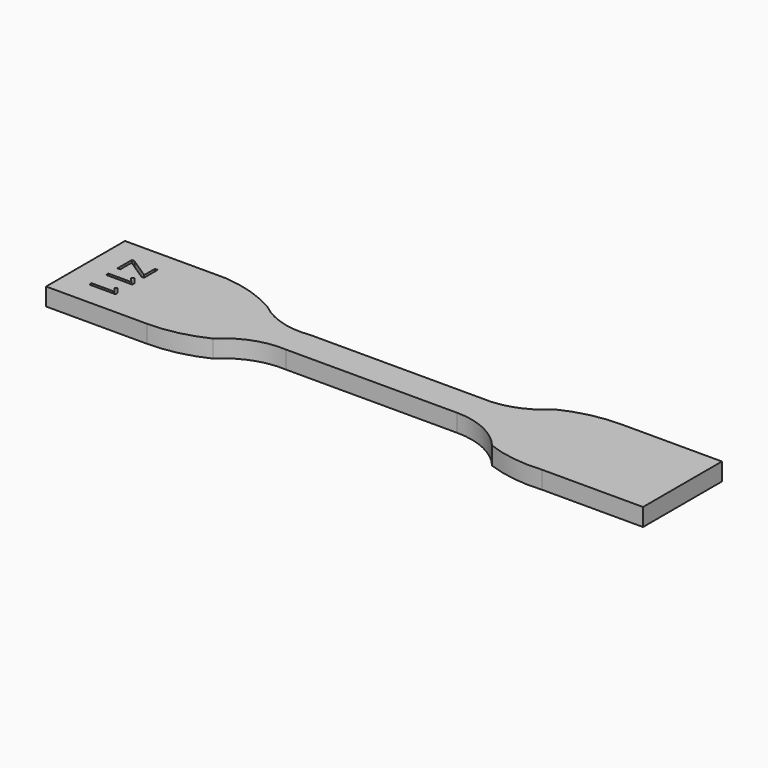
from build123d import *

# Parameters (mm, degrees)
F1_DEPTH     = 3.4
F2_TEXT_SIZE = 7.0564552314
F3_DEPTH     = 1


# Not quite as in the source:
# - Text() gives the source's letters only with a copy of the font that has no kerning and outlines rounded to 1/6400 em; it was checked with that copy


with BuildPart() as f1:
    # F0 (on Top) → F1 (new body)
    with BuildSketch(Plane.XY):
        with BuildLine():
            Line((-14.4320548165, 19.7811394548), (-33.8720548165, 19.7811394548))
            Line((-33.8720548165, 19.7811394548), (-33.8720548165, 0.7811394548))
            Line((-33.8720548165, 0.7811394548), (-14.4320548165, 0.7811394548))
            ThreePointArc((-14.4320548165, 0.7811394548), (-8.9053122052, 1.3996892086), (-3.6520548165, 3.2247301661))
            ThreePointArc((-3.6520548165, 3.2247301661), (1.3014698263, 6.4128780055), (7.1279451835, 7.2811394548))
            Line((7.1279451835, 7.2811394548), (40.1279451835, 7.2811394548))
            ThreePointArc((40.1279451835, 7.2811394548), (46.0837574042, 5.9511158081), (50.9079451835, 2.2137538538))
            ThreePointArc((50.9079451835, 2.2137538538), (56.2191047011, 0.9041953221), (61.6879451835, 0.7811394548))
            Line((61.6879451835, 0.7811394548), (81.1279451835, 0.7811394548))
            Line((81.1279451835, 0.7811394548), (81.1279451835, 19.7811394548))
            Line((81.1279451835, 19.7811394548), (61.6879451835, 19.7811394548))
            ThreePointArc((61.6879451835, 19.7811394548), (56.1612025723, 19.162589701), (50.9079451835, 17.3375487435))
            ThreePointArc((50.9079451835, 17.3375487435), (45.9544205407, 14.1494009041), (40.1279451835, 13.2811394548))
            Line((40.1279451835, 13.2811394548), (7.1279451835, 13.2811394548))
            ThreePointArc((7.1279451835, 13.2811394548), (1.4167452884, 13.6925537245), (-3.6520548165, 16.3560723447))
            ThreePointArc((-3.6520548165, 16.3560723447), (-8.8458057958, 18.686276846), (-14.4320548165, 19.7811394548))
        make_face()
    extrude(amount=F1_DEPTH)

    # F2 (on face) → F3 (cut)
    with BuildSketch(Plane.XY.offset(3.4)):
        with Locations(Location((-29.1824135929, 15.8650862949), (0, 0, -90))):
            Text('Z11', F2_TEXT_SIZE, font='Open Sans', text_align=(TextAlign.LEFT, TextAlign.BOTTOM))
    extrude(amount=-F3_DEPTH, mode=Mode.SUBTRACT)


solid = f1.part
